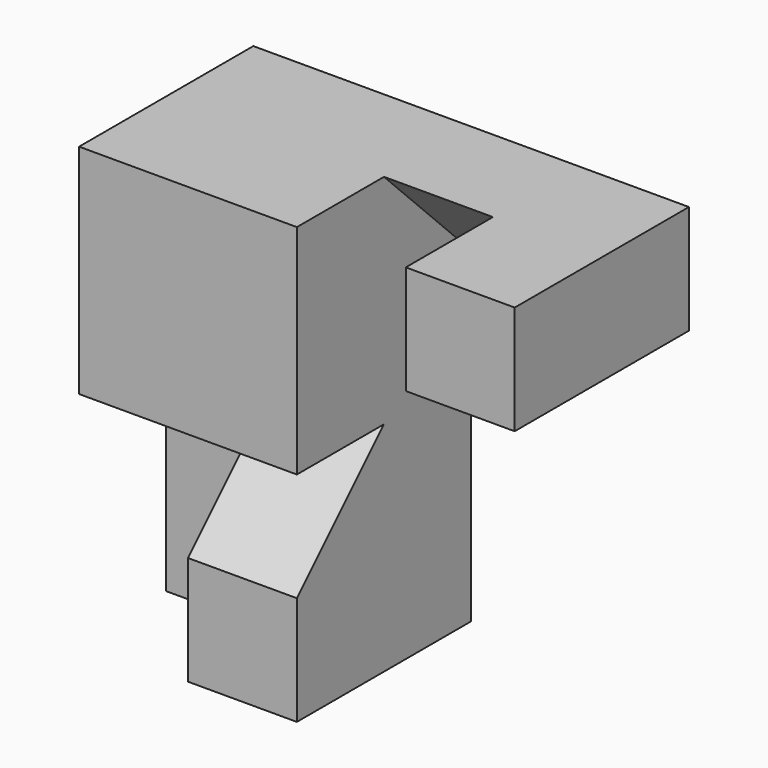
from build123d import *

# Parameters (mm, degrees)
F0_W      = 8
F0_H      = 8
F1_DEPTH  = 8
F2_DEPTH  = 16
F4_DEPTH  = 8
F5_DEPTH  = 16
F0_W_2    = 16
F0_H_2    = 16
F6_DEPTH  = 8
F7_W      = 8
F7_H      = 16
F8_DEPTH  = 8
F10_DEPTH = 8


with BuildPart() as f1:
    # F0 (on Front) → F1 (new body)
    with BuildSketch(Plane.XZ):
        with Locations((-40.0961564034, 37.5077876064)):
            Rectangle(F0_W, F0_H)
    extrude(amount=F1_DEPTH)

    # F0 (on Front) → F2 (join)
    with BuildSketch(Plane.XZ):
        Polygon((-44.0961564034, 41.5077876064), (-60.0961564034, 41.5077876064), (-60.0961564034, 25.5077876064), (-44.0961564034, 25.5077876064), (-44.0961564034, 33.5077876064), align=None)
    extrude(amount=F2_DEPTH)

    # F3 (on face) → F4 (cut)
    with BuildSketch(Plane.YZ.offset(-36.0961564034)):
        Polygon((0, 33.5077876064), (-8, 41.5077876064), (-8, 33.5077876064), align=None)
    extrude(amount=-F4_DEPTH, mode=Mode.SUBTRACT)

    # F0 (on Front) → F5 (join)
    with BuildSketch(Plane.XZ):
        with Locations((-32.0961564034, 37.5077876064)):
            Rectangle(F0_W, F0_H)
    extrude(amount=F5_DEPTH)

    # F0 (on Front) → F6 (join)
    with BuildSketch(Plane.XZ):
        with Locations((-52.0961564034, 17.5077876064)):
            Rectangle(F0_W_2, F0_H_2)
    extrude(amount=F6_DEPTH)

    # F7 (on face) → F8 (join)
    with BuildSketch(Plane.XZ.offset(8)):
        with Locations((-48.0961564034, 17.5077876064)):
            Rectangle(F7_W, F7_H)
    extrude(amount=F8_DEPTH)

    # F9 (on face) → F10 (cut)
    with BuildSketch(Plane(origin=(-52.0961564034, 0, 0), x_dir=(0, -1, 0), z_dir=(-1, 0, 0))):
        Polygon((8, 25.5077876064), (16, 17.5077876064), (16, 25.5077876064), align=None)
    extrude(amount=-F10_DEPTH, mode=Mode.SUBTRACT)


solid = f1.part
